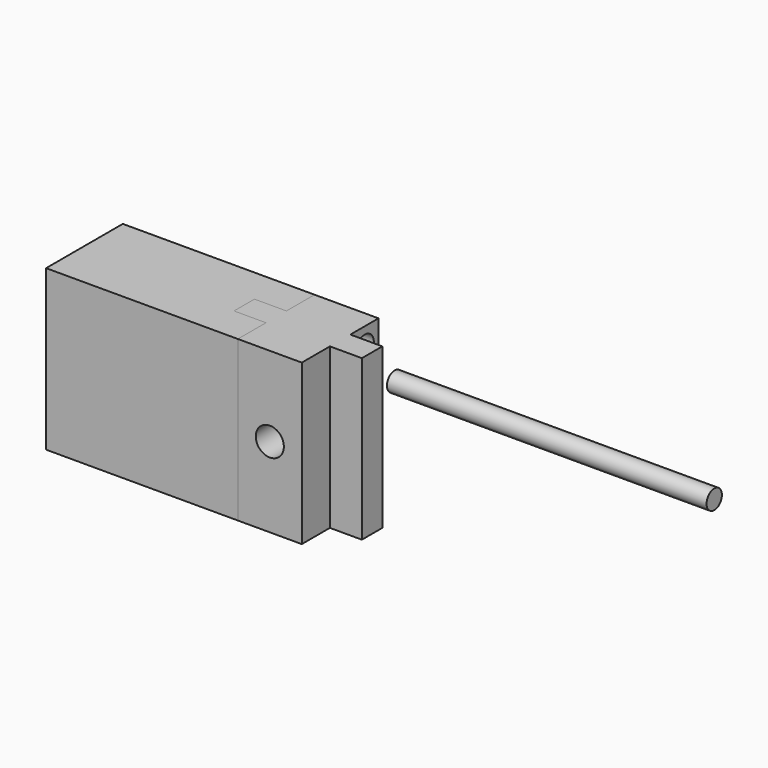
from build123d import *

# Parameters (mm, degrees)
F0_W      = 30
F0_H      = 15
F1_DEPTH  = 25
F2_W      = 5
F2_H      = 4
F3_DEPTH  = 25.001
F5_DEPTH  = 25
F6_R      = 1.75
F7_DEPTH  = 45.001
F8_R      = 1.75
F9_DEPTH  = 40.001
F10_R     = 1.5
F11_DEPTH = 50
F13_D     = 4.4


# Not quite as in the source:
# - a feature names something its author has since deleted; it is built from what else it names


with BuildPart() as f1:
    # F0 (on Top) → F1 (new body)
    with BuildSketch(Plane.XY):
        with Locations((-36.4950267971, -24.0964780748)):
            Rectangle(F0_W, F0_H)
    extrude(amount=F1_DEPTH)

    # F2 (on face) → F3 (cut, through all)
    with BuildSketch(Plane.XY.offset(25)):
        with Locations((-23.9950267971, -24.0964780748)):
            Rectangle(F2_W, F2_H)
    extrude(amount=-F3_DEPTH, mode=Mode.SUBTRACT)


with BuildPart() as f5:
    # F4 (on face) → F5 (new body)
    with BuildSketch(Plane.XY.offset(25)):
        Polygon((-11.4950267971, -16.5964780748), (-21.4950267971, -16.5964780748), (-21.4950267971, -22.0964780748), (-26.4950267971, -22.0964780748), (-26.4950267971, -26.0964780748), (-21.4950267971, -26.0964780748), (-21.4950267971, -31.5964780748), (-11.4950267971, -31.5964780748), (-11.4950267971, -26.0964780748), (-6.4950267971, -26.0964780748), (-6.4950267971, -22.0964780748), (-11.4950267971, -22.0964780748), align=None)
    extrude(amount=-F5_DEPTH)


with BuildPart() as f7_tool:
    # F6 (on face) → F7 (new body, through all)
    with BuildSketch(Plane(origin=(-51.4950267971, 0, 0), x_dir=(0, -1, 0), z_dir=(-1, 0, 0))):
        with Locations((19.3429368734, 13.1029868498)):
            Circle(F6_R)
    extrude(amount=-F7_DEPTH)


with BuildPart() as f1_1:
    add(f1.part)

    # F7: cut by f7_tool
    add(f7_tool.part, mode=Mode.SUBTRACT)


with BuildPart() as f5_1:
    add(f5.part)

    # F7: cut by f7_tool
    add(f7_tool.part, mode=Mode.SUBTRACT)

    # F8 (on face) → F9 (cut, through all)
    with BuildSketch(Plane.YZ.offset(-11.4950267971)):
        with Locations((-19.257010007, 22.1025766501)):
            Circle(F8_R)
        with Locations((-19.2999734402, 17.60278175)):
            Circle(F8_R)
        with Locations((-19.3829028493, 8.6031643288)):
            Circle(F8_R)
        with Locations((-19.4228688251, 4.1033418078)):
            Circle(F8_R)
    extrude(amount=-F9_DEPTH, mode=Mode.SUBTRACT)

    # F13 (through all)
    with Locations(Plane.XZ.offset(31.5964780748)):
        with Locations((-16.4950267971, 12.5)):
            Hole(F13_D / 2)


with BuildPart() as f11:
    # F10 (on face) → F11 (new body)
    with BuildSketch(Plane.YZ.offset(-11.4950267971)):
        with Locations((-13.4415747598, 15.0504745543)):
            Circle(F10_R)
    extrude(amount=F11_DEPTH)


solid = Compound([f1_1.part, f5_1.part, f11.part])
